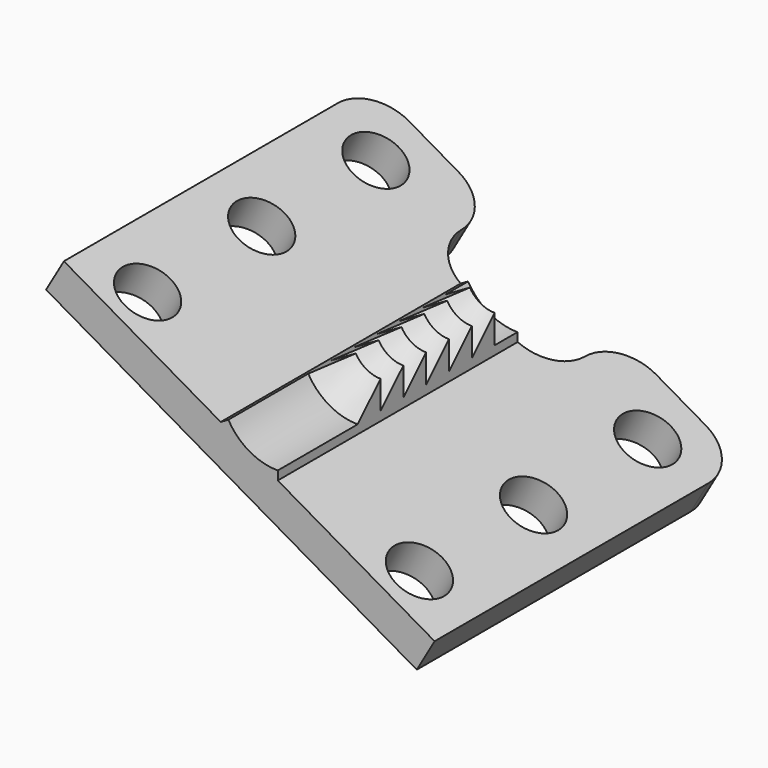
from build123d import *

# Parameters (mm, degrees)
F1_ANGLE = 60
F3_DEPTH = 27
F4_R     = 2
F5_DEPTH = 15.4913810568
F6_W     = 10
F6_H     = 6
F7_DEPTH = 15.4913810568
F8_R     = 2.99999


# Not quite as in the source:
# - a fillet or chamfer is up to 0.001 mm smaller than in the source, because OpenCascade refuses the exact size


with BuildPart() as f1:
    # F0 (on Right) → F1 (revolve)
    with BuildSketch(Plane.YZ):
        Polygon((7, 0), (0, 0), (0, -2.5), (26, -2.5), (26, 0), (19, 0), (19, 2), (17, 0), (17, 2), (15, 0), (15, 2), (13, 0), (13, 2), (11, 0), (11, 2), (9, 0), (9, 2), align=None)
    revolve(axis=Axis((0, 13.3030909821, 4), (0, 1, 0)), revolution_arc=F1_ANGLE)

    # F2 (on face) → F3 (join)
    with BuildSketch(Plane.XZ):
        Polygon((10.9903810568, -6.9641016151), (-2, 0.5358983849), (-3.25, -1.6291651246), (9.7403810568, -9.1291651246), align=None)
        Polygon((-3.25, -1.6291651246), (-2, 0.5358983849), (-14.9903810568, 8.0358983849), (-16.2403810568, 5.8708348754), align=None)
    extrude(amount=-F3_DEPTH)

    # F4 (on face) → F5 (cut, through all)
    with BuildSketch(Plane(origin=(-1.5179491924, 0, -2.6291651246), x_dir=(0.8660254038, 0, -0.5), z_dir=(-0.5, 0, -0.8660254038))):
        with Locations((-13, -3)):
            Circle(F4_R)
        with Locations((9, -3)):
            Circle(F4_R)
        with Locations((-13, -13)):
            Circle(F4_R)
        with Locations((9, -13)):
            Circle(F4_R)
        with Locations((-13, -23)):
            Circle(F4_R)
        with Locations((9, -23)):
            Circle(F4_R)
    extrude(amount=-F5_DEPTH, mode=Mode.SUBTRACT)

    # F6 (on face) → F7 (cut, through all)
    with BuildSketch(Plane(origin=(-1.5179491924, 0, -2.6291651246), x_dir=(0.8660254038, 0, -0.5), z_dir=(-0.5, 0, -0.8660254038))):
        with Locations((-2, -24)):
            Rectangle(F6_W, F6_H)
    extrude(amount=-F7_DEPTH, mode=Mode.SUBTRACT)

    # F8 (radius 3 in the source; OpenCascade refuses exactly that, so slightly less here)
    f8_edges = [f1.edges().sort_by_distance(p)[0] for p in [
        (1.705127, 21, -3.046633),
        (1.705127, 27, -3.046633),
        (-6.955127, 27, 1.953367),
        (-6.955127, 21, 1.953367),
        (-15.615381, 27, 6.953367),
        (10.365381, 27, -8.046633),
    ]]
    fillet(f8_edges, radius=F8_R)


solid = f1.part
